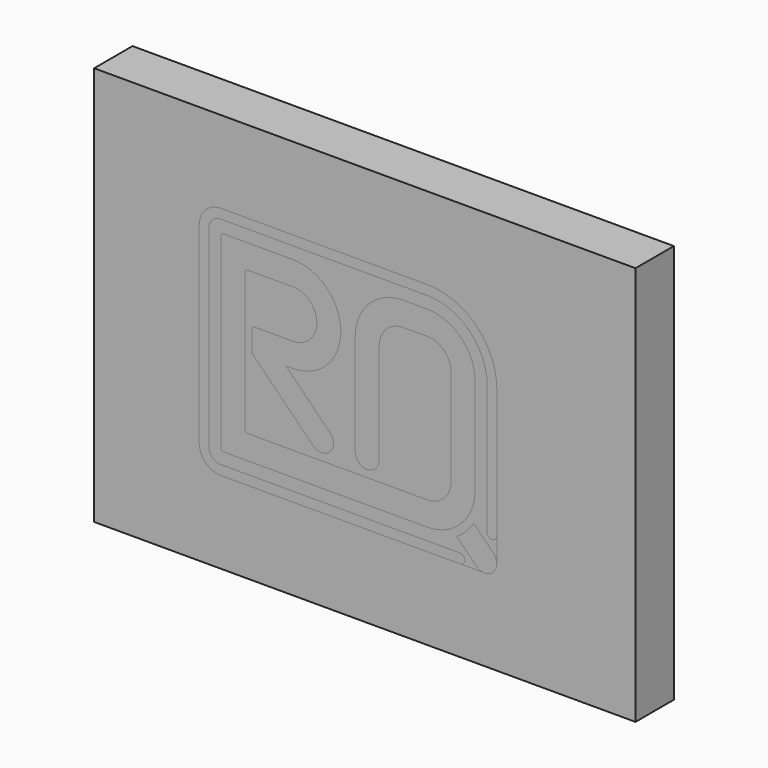
from build123d import *

# Parameters (mm, degrees)
F1_DEPTH = 10
F2_DEPTH = 10
F0_W     = 112.8634214401
F0_H     = 83.2712948322
F4_DEPTH = 10


# Not quite as in the source:
# - ends of sketch curves that miss each other by under 0.0002 mm in the source are joined
# - a feature of the source that left no trace in its solid (it failed there, or was rolled back) is left out
# - a feature names something its author has since deleted; it is built from what else it names


with BuildPart() as f1:
    # F0 (on Front) → F1 (new body)
    with BuildSketch(Plane.XZ):
        with BuildLine():
            Line((-25, -14.4999996647), (-25, 14.5))
            ThreePointArc((-25, 14.5), (-24.8535533906, 14.8535533906), (-24.5, 15))
            Line((-24.5, 15), (-15, 15))
            ThreePointArc((-15, 15), (-11.493877298, 13.5647024558), (-10.0006863175, 10.0828414395))
            ThreePointArc((-10.0006863175, 10.0828414395), (-11.4352975442, 6.493877298), (-15, 5))
            Line((-15, 5), (-23, 5))
            ThreePointArc((-23, 5), (-23.3535533906, 4.8535533906), (-23.5, 4.5))
            Line((-23.5, 4.5), (-23.5, 0.2061669839))
            ThreePointArc((-23.5, 0.2061669839), (-23.4887525914, 0.1007112853), (-23.4555163825, 0))
            Line((-23.4555163825, 0), (-16.4515272404, 0))
            Line((-16.4515272404, 0), (-15, 0))
            ThreePointArc((-15, 0), (-8.0470582749, 2.8127473004), (-5.0054901633, 9.6686797265))
            Line((-5.0054901633, 9.6686797265), (-5.0054901633, 10.3313202735))
            ThreePointArc((-5.0054901633, 10.3313202735), (-8.0470582749, 17.1872526996), (-15, 20))
            Line((-15, 20), (-25, 20))
            Line((-25, 20), (-29.5000011921, 20))
            ThreePointArc((-29.5000011921, 20), (-29.8535545827, 19.8535533906), (-30.0000011921, 19.5))
            Line((-30.0000011921, 19.5), (-30.0000011921, 17.5))
            Line((-30.0000011921, 17.5), (-30.0000011921, -19.5))
            ThreePointArc((-30.0000011921, -19.5), (-29.8535545827, -19.8535533906), (-29.5000011921, -20))
            Line((-29.5000011921, -20), (-25, -20))
            Line((-25, -20), (-2.0054901633, -20))
            Line((-2.0054901633, -20), (-0.3755952516, -20))
            Line((-0.3755952516, -20), (8.9945098367, -20))
            Line((8.9945098367, -20), (12.9945098367, -20))
            ThreePointArc((12.9945098367, -20), (20.0655776486, -17.0710678119), (22.9945098367, -10))
            Line((22.9945098367, -10), (22.9945098367, 10))
            ThreePointArc((22.9945098367, 10), (20.0655776486, 17.0710678119), (12.9945098367, 20))
            Line((12.9945098367, 20), (7.9945098367, 20))
            ThreePointArc((7.9945098367, 20), (0.9234420249, 17.0710678119), (-2.0054901633, 10))
            Line((-2.0054901633, 10), (-2.0054901633, -11.0000000643))
            ThreePointArc((-2.0054901633, -11.0000000643), (-1.2732571162, -12.7677670173), (0.4945098367, -13.5000000643))
            ThreePointArc((0.4945098367, -13.5000000643), (2.262277125, -12.7677670173), (2.994510172, -11.0000000643))
            Line((2.994510172, -11.0000000643), (2.994510172, 10))
            ThreePointArc((2.994510172, 10), (4.4589761679, 13.5355336689), (7.9945098367, 14.9999996647))
            Line((7.9945098367, 14.9999996647), (12.9945098367, 14.9999996647))
            ThreePointArc((12.9945098367, 14.9999996647), (16.5300435056, 13.5355336689), (17.9945095014, 10))
            Line((17.9945095014, 10), (17.9945095014, -10))
            ThreePointArc((17.9945095014, -10), (16.9612762133, -13.0438070177), (14.2886047885, -14.8296288577))
            ThreePointArc((14.2886047885, -14.8296288577), (13.6471406581, -14.9572239871), (12.9945098367, -14.9999996647))
            Line((12.9945098367, -14.9999996647), (8.9945098367, -14.9999996647))
            Line((8.9945098367, -14.9999996647), (-0.0054901633, -15.0000000878))
            Line((-0.0054901633, -15.0000000878), (-0.3755952516, -15.0000001052))
            Line((-0.3755952516, -15.0000001052), (-1.0054901633, -15.0000001348))
            Line((-1.0054901633, -15.0000001348), (-24.5, -14.9999996647))
            ThreePointArc((-24.5, -14.9999996647), (-24.8535533906, -14.8535530553), (-25, -14.4999996647))
        make_face()
        with BuildLine():
            Line((-16.4515272404, 0), (-23.4555163825, 0))
            ThreePointArc((-23.4555163825, 0), (-23.4116485183, -0.0776384025), (-23.3546867552, -0.1462493971))
            Line((-23.3546867552, -0.1462493971), (-10.8196093867, -12.7620815701))
            ThreePointArc((-10.8196093867, -12.7620815701), (-9.0542025953, -13.4999867782), (-7.284093705, -12.773433441))
            ThreePointArc((-7.284093705, -12.773433441), (-6.5461885926, -11.0080267446), (-7.2727419298, -9.2379178544))
            Line((-7.2727419298, -9.2379178544), (-16.4515272404, 0))
        make_face()
    extrude(amount=-F1_DEPTH)


with BuildPart() as f1b:
    # F0 (on Front) → F1, piece 2 (new body)
    with BuildSketch(Plane.XZ):
        with BuildLine():
            ThreePointArc((22.6995307229, -16.1694869802), (21.1262378204, -18.1317279836), (19.163996817, -19.7050208862))
            Line((19.163996817, -19.7050208862), (21.979791211, -22.5208152802))
            Line((21.979791211, -22.5208152802), (23.2475581639, -23.7885822331))
            ThreePointArc((23.2475581639, -23.7885822331), (24.058616536, -24.3305141114), (25.0153251169, -24.5208152802))
            ThreePointArc((25.0153251169, -24.5208152802), (26.7603747249, -23.8110113213), (27.5145098367, -22.0846567728))
            Line((27.5145098367, -22.0846567728), (27.5145098367, -21.9569737876))
            ThreePointArc((27.5145098367, -21.9569737876), (27.3126190985, -21.0346913722), (26.7830920699, -20.2530483272))
            Line((26.7830920699, -20.2530483272), (25.5145098367, -18.9844660941))
            Line((25.5145098367, -18.9844660941), (22.6995307229, -16.1694869802))
        make_face()
    extrude(amount=-F1_DEPTH)


with BuildPart() as f1c:
    # F0 (on Front) → F1, piece 3 (new body)
    with BuildSketch(Plane.XZ):
        with BuildLine():
            ThreePointArc((20.8512915522, -23.5208161175), (20.5609319978, -22.816252112), (19.8584706764, -22.5208418878))
            ThreePointArc((19.8584706764, -22.5208418878), (18.8512979948, -23.5172265323), (19.8512915522, -24.5208161175))
            ThreePointArc((19.8512915522, -24.5208161175), (20.5583983334, -24.2279228987), (20.8512915522, -23.5208161175))
        make_face()
        with BuildLine():
            Line((-30.0200011921, -24.5208152802), (19.8512915522, -24.5208152802))
            ThreePointArc((19.8512915522, -24.5208152802), (18.8512979948, -23.5172265323), (19.8584706764, -22.5208418878))
            Line((19.8584706764, -22.5208418878), (-30.0200011921, -22.5208152802))
            ThreePointArc((-30.0200011921, -22.5208152802), (-31.7877681451, -21.7885822331), (-32.5200011921, -20.0208152802))
            Line((-32.5200011921, -20.0208152802), (-32.5200011921, 20.02))
            ThreePointArc((-32.5200011921, 20.02), (-31.7877681451, 21.787766953), (-30.0200011921, 22.52))
            Line((-30.0200011921, 22.52), (12.9945098367, 22.52))
            ThreePointArc((12.9945098367, 22.52), (21.8474867372, 18.8529769005), (25.5145098367, 10))
            Line((25.5145098367, 10), (25.5145098367, -16.8946627527))
            ThreePointArc((25.5145098367, -16.8946627527), (26.5145098367, -15.8946627527), (27.5145098367, -16.8946627527))
            Line((27.5145098367, -16.8946627527), (27.5145098367, 10))
            ThreePointArc((27.5145098367, 10), (23.2617002996, 20.2671904628), (12.9945098367, 24.52))
            Line((12.9945098367, 24.52), (-30.0200011921, 24.52))
            ThreePointArc((-30.0200011921, 24.52), (-33.2019817074, 23.2019805153), (-34.5200011921, 20.02))
            Line((-34.5200011921, 20.02), (-34.5200011921, -20.0208152802))
            ThreePointArc((-34.5200011921, -20.0208152802), (-33.2019817074, -23.2027957955), (-30.0200011921, -24.5208152802))
        make_face()
        with BuildLine():
            ThreePointArc((26.5145098367, -17.8946627527), (27.2216166179, -17.6017695339), (27.5145098367, -16.8946627527))
            ThreePointArc((27.5145098367, -16.8946627527), (26.5145098367, -15.8946627527), (25.5145098367, -16.8946627527))
            ThreePointArc((25.5145098367, -16.8946627527), (25.8074030555, -17.6017695339), (26.5145098367, -17.8946627527))
        make_face()
    extrude(amount=-F1_DEPTH)


with BuildPart() as f2:
    # F0 (on Front) → F2 (new body)
    with BuildSketch(Plane.XZ):
        with BuildLine():
            Line((21.979791211, -22.5208152802), (19.163996817, -19.7050208862))
            ThreePointArc((19.163996817, -19.7050208862), (21.1262378204, -18.1317279836), (22.6995307229, -16.1694869802))
            Line((22.6995307229, -16.1694869802), (25.5145098367, -18.9844660941))
            Line((25.5145098367, -18.9844660941), (26.7830920699, -20.2530483272))
            ThreePointArc((26.7830920699, -20.2530483272), (27.3126190985, -21.0346913722), (27.5145098367, -21.9569737876))
            Line((27.5145098367, -21.9569737876), (27.5145098367, -18.8631457505))
            Line((27.5145098367, -18.8631457505), (27.5145098367, -16.8946627527))
            ThreePointArc((27.5145098367, -16.8946627527), (27.2216166179, -17.6017695339), (26.5145098367, -17.8946627527))
            ThreePointArc((26.5145098367, -17.8946627527), (25.8074030555, -17.6017695339), (25.5145098367, -16.8946627527))
            Line((25.5145098367, -16.8946627527), (25.5145098367, 10))
            ThreePointArc((25.5145098367, 10), (21.8474867372, 18.8529769005), (12.9945098367, 22.52))
            Line((12.9945098367, 22.52), (-30.0200011921, 22.52))
            ThreePointArc((-30.0200011921, 22.52), (-31.7877681451, 21.787766953), (-32.5200011921, 20.02))
            Line((-32.5200011921, 20.02), (-32.5200011921, -20.0208152802))
            ThreePointArc((-32.5200011921, -20.0208152802), (-31.7877681451, -21.7885822331), (-30.0200011921, -22.5208152802))
            Line((-30.0200011921, -22.5208152802), (19.8584708674, -22.5208152802))
            ThreePointArc((19.8584708674, -22.5208152802), (20.5609319978, -22.816252112), (20.8512915522, -23.5208161175))
            ThreePointArc((20.8512915522, -23.5208161175), (20.5583983334, -24.2279228987), (19.8512915522, -24.5208161175))
            Line((19.8512915522, -24.5208161175), (21.8584708674, -24.5208152802))
            Line((21.8584708674, -24.5208152802), (25.0153251169, -24.5208152802))
            ThreePointArc((25.0153251169, -24.5208152802), (24.058616536, -24.3305141114), (23.2475581639, -23.7885822331))
            Line((23.2475581639, -23.7885822331), (21.979791211, -22.5208152802))
        make_face()
        with BuildLine():
            Line((-25, 20), (-15, 20))
            Line((-15, 20), (7.9945098367, 20))
            Line((7.9945098367, 20), (12.9945098367, 20))
            ThreePointArc((12.9945098367, 20), (20.0655776486, 17.0710678119), (22.9945098367, 10))
            Line((22.9945098367, 10), (22.9945098367, -10))
            ThreePointArc((22.9945098367, -10), (20.0655776486, -17.0710678119), (12.9945098367, -20))
            Line((12.9945098367, -20), (8.9945098367, -20))
            Line((8.9945098367, -20), (-0.3755952516, -20))
            Line((-0.3755952516, -20), (-2.0054901633, -20))
            Line((-2.0054901633, -20), (-25, -20))
            Line((-25, -20), (-29.5000011921, -20))
            ThreePointArc((-29.5000011921, -20), (-29.8535545827, -19.8535533906), (-30.0000011921, -19.5))
            Line((-30.0000011921, -19.5), (-30.0000011921, 17.5))
            Line((-30.0000011921, 17.5), (-30.0000011921, 19.5))
            ThreePointArc((-30.0000011921, 19.5), (-29.8535545827, 19.8535533906), (-29.5000011921, 20))
            Line((-29.5000011921, 20), (-25, 20))
        make_face(mode=Mode.SUBTRACT)
        with BuildLine():
            ThreePointArc((-24.5, 15), (-24.8535533906, 14.8535533906), (-25, 14.5))
            Line((-25, 14.5), (-25, -14.4999996647))
            ThreePointArc((-25, -14.4999996647), (-24.8535533906, -14.8535530553), (-24.5, -14.9999996647))
            Line((-24.5, -14.9999996647), (-1.0054901633, -14.9999996647))
            Line((-1.0054901633, -14.9999996647), (-0.3755952516, -15.0000001348))
            Line((-0.3755952516, -15.0000001348), (-0.0054901633, -15.0000000878))
            Line((-0.0054901633, -15.0000000878), (8.9945098367, -14.9999996647))
            Line((8.9945098367, -14.9999996647), (12.9945098367, -14.9999996647))
            ThreePointArc((12.9945098367, -14.9999996647), (13.6471406581, -14.9572239871), (14.2886047885, -14.8296288577))
            ThreePointArc((14.2886047885, -14.8296288577), (16.9612762133, -13.0438070177), (17.9945095014, -10))
            Line((17.9945095014, -10), (17.9945095014, 10))
            ThreePointArc((17.9945095014, 10), (16.5300435056, 13.5355336689), (12.9945098367, 14.9999996647))
            Line((12.9945098367, 14.9999996647), (7.9945098367, 14.9999996647))
            ThreePointArc((7.9945098367, 14.9999996647), (4.4589761679, 13.5355336689), (2.994510172, 10))
            Line((2.994510172, 10), (2.994510172, -11.0000000643))
            ThreePointArc((2.994510172, -11.0000000643), (2.262277125, -12.7677670173), (0.494510172, -13.5000000643))
            ThreePointArc((0.494510172, -13.5000000643), (-1.2732571162, -12.7677670173), (-2.0054901633, -11.0000000643))
            Line((-2.0054901633, -11.0000000643), (-2.0054901633, 10))
            ThreePointArc((-2.0054901633, 10), (0.9234420249, 17.0710678119), (7.9945098367, 20))
            Line((7.9945098367, 20), (-15, 20))
            ThreePointArc((-15, 20), (-8.0470582749, 17.1872526996), (-5.0054901633, 10.3313202735))
            ThreePointArc((-5.0054901633, 10.3313202735), (-5, 10), (-5.0054901633, 9.6686797265))
            ThreePointArc((-5.0054901633, 9.6686797265), (-8.0470582749, 2.8127473004), (-15, 0))
            Line((-15, 0), (-16.4515272404, 0))
            Line((-16.4515272404, 0), (-7.2727419298, -9.2379178544))
            ThreePointArc((-7.2727419298, -9.2379178544), (-6.5461885926, -11.0080267446), (-7.2840938007, -12.773433536))
            ThreePointArc((-7.2840938007, -12.773433536), (-9.0542025953, -13.4999867782), (-10.8196093867, -12.7620815701))
            Line((-10.8196093867, -12.7620815701), (-23.3546867552, -0.1462493971))
            ThreePointArc((-23.3546867552, -0.1462493971), (-23.4116485183, -0.0776384025), (-23.4555163825, 0))
            ThreePointArc((-23.4555163825, 0), (-23.4887525914, 0.1007112853), (-23.5, 0.2061669839))
            Line((-23.5, 0.2061669839), (-23.5, 4.5))
            ThreePointArc((-23.5, 4.5), (-23.3535533906, 4.8535533906), (-23, 5))
            Line((-23, 5), (-15, 5))
            ThreePointArc((-15, 5), (-11.4352975442, 6.493877298), (-10.0006863175, 10.0828414395))
            ThreePointArc((-10.0006863175, 10.0828414395), (-11.493877298, 13.5647024558), (-15, 15))
            Line((-15, 15), (-24.5, 15))
        make_face()
    extrude(amount=-F2_DEPTH)


with BuildPart() as f4:
    # F0 (on Front) → F4 (new body)
    with BuildSketch(Plane.XZ):
        Rectangle(F0_W, F0_H)
        with BuildLine():
            ThreePointArc((27.5145098367, -22.0846567728), (26.7603747249, -23.8110113213), (25.0153251169, -24.5208152802))
            Line((25.0153251169, -24.5208152802), (21.8584708674, -24.5208152802))
            Line((21.8584708674, -24.5208152802), (19.8512915522, -24.5208152802))
            Line((19.8512915522, -24.5208152802), (-30.0200011921, -24.5208152802))
            ThreePointArc((-30.0200011921, -24.5208152802), (-33.2019817074, -23.2027957955), (-34.5200011921, -20.0208152802))
            Line((-34.5200011921, -20.0208152802), (-34.5200011921, 20.02))
            ThreePointArc((-34.5200011921, 20.02), (-33.2019817074, 23.2019805153), (-30.0200011921, 24.52))
            Line((-30.0200011921, 24.52), (12.9945098367, 24.52))
            ThreePointArc((12.9945098367, 24.52), (23.2617002996, 20.2671904628), (27.5145098367, 10))
            Line((27.5145098367, 10), (27.5145098367, -16.8946627527))
            Line((27.5145098367, -16.8946627527), (27.5145098367, -18.8631457505))
            Line((27.5145098367, -18.8631457505), (27.5145098367, -21.9569737876))
            ThreePointArc((27.5145098367, -21.9569737876), (27.5153251169, -22.0208152802), (27.5145098367, -22.0846567728))
        make_face(mode=Mode.SUBTRACT)
    extrude(amount=-F4_DEPTH)


solid = Compound([f1.part, f1b.part, f1c.part, f2.part, f4.part])
